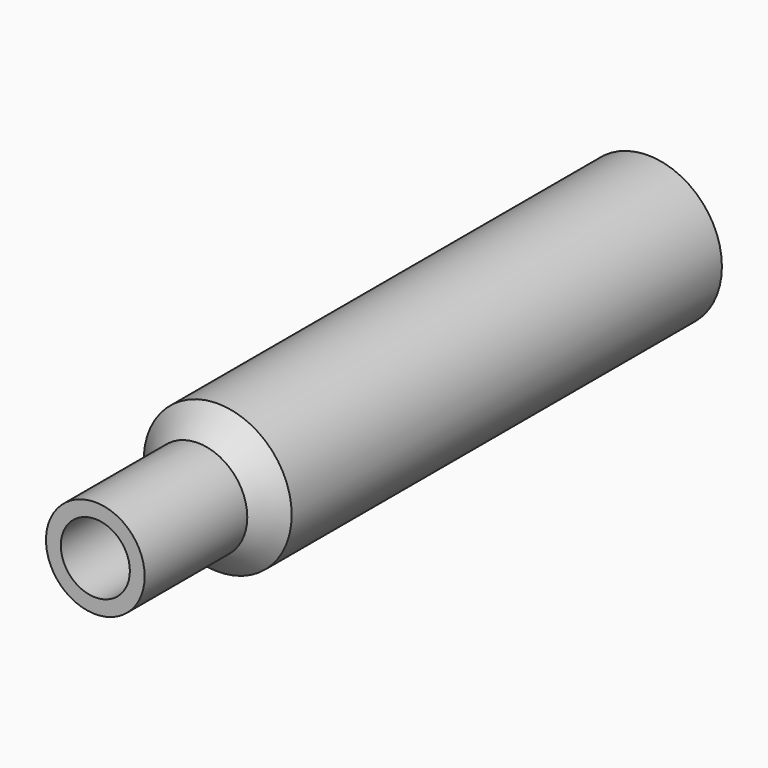
from build123d import *

# Parameters (mm, degrees)
F0_R        = 0.75
F1_DEPTH    = 2.2
F2_DEPTH    = 3.5
F3_R        = 0.55
F4_DEPTH    = 5
F5_R        = 0.35
F6_DEPTH    = 5
F7_S5_R     = 0.35
F7_T6_DEPTH = 2
F8_R        = 0.5
F8_R_2      = 0.35
F9_DEPTH    = 1.3
F10_SIZE    = 0.24999


# Not quite as in the source:
# - a fillet or chamfer that OpenCascade refuses, or shapes differently, is made with other operations: its cross-section is extruded or revolved along the edge and cut away or added
# - a fillet or chamfer is up to 0.001 mm smaller than in the source, because OpenCascade refuses the exact size


with BuildPart() as f1:
    # F0 (on Front) → F1 (new body)
    with BuildSketch(Plane.XZ):
        Circle(F0_R)
    extrude(amount=F1_DEPTH)

    # F2 (add): a face of the model
    f2_faces = [f1.faces().sort_by_distance(p)[0] for p in [
        (0, 0, 0),
    ]]
    extrude(f2_faces, amount=F2_DEPTH)

    # F3 (on Front) → F4 (cut)
    with BuildSketch(Plane.XZ):
        Circle(F3_R)
    extrude(amount=-F4_DEPTH, mode=Mode.SUBTRACT)

    # F5 (on Front) → F6 (cut)
    with BuildSketch(Plane.XZ):
        Circle(F5_R)
    extrude(amount=F6_DEPTH, mode=Mode.SUBTRACT)

    # F7: chamfer of 0.25 on 1 edges, made by hand


with BuildPart() as f7_tool2:
    # F7_s3 → F7_t4 (revolve)
    with BuildSketch(Plane.XY):
        Polygon((0.55, 0.25), (0.3, 0), (0.55, 0), align=None)
    revolve(axis=Axis((0, 0, 0), (0, -1, 0)))

    # F7_s5 → F7_t6 (cut, symmetric)
    with BuildSketch(Plane.XZ.offset(-0.1)):
        Circle(F7_S5_R)
    extrude(amount=F7_T6_DEPTH, both=True, mode=Mode.SUBTRACT)


with BuildPart() as f1_1:
    add(f1.part)

    # F7_t1: union F7_tool2
    add(f7_tool2.part)

    # F8 (on face) → F9 (join)
    with BuildSketch(Plane.XZ.offset(2.2)):
        Circle(F8_R)
        Circle(F8_R_2, mode=Mode.SUBTRACT)
    extrude(amount=F9_DEPTH)

    # F10 (size 0.25 in the source; OpenCascade refuses exactly that, so slightly less here)
    f10_edges = [f1_1.edges().sort_by_distance(p)[0] for p in [
        (-0.75, -2.2, 0),
    ]]
    chamfer(f10_edges, length=F10_SIZE)


solid = f1_1.part
